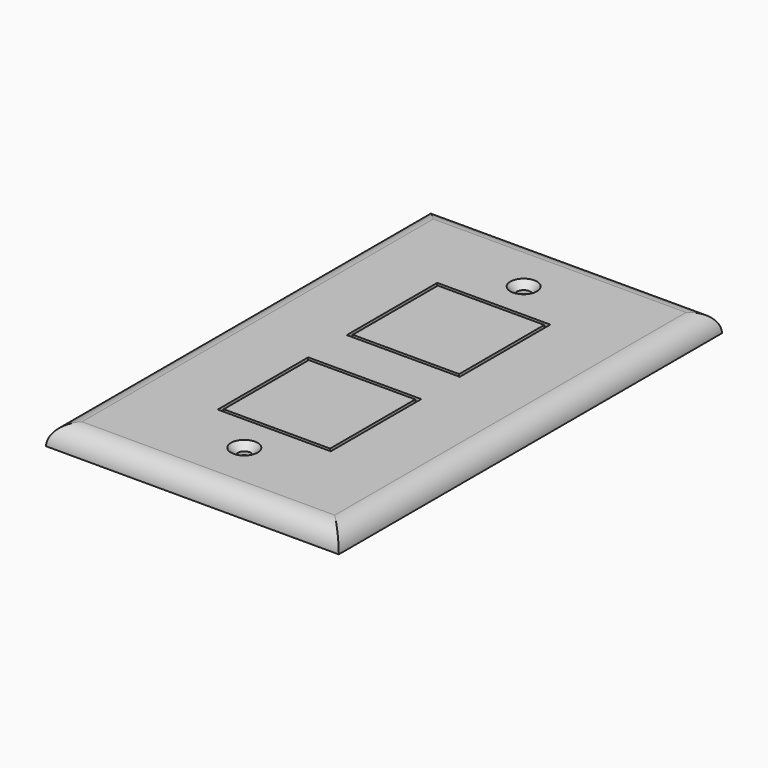
from build123d import *

# Parameters (mm, degrees)
F0_W        = 69.85
F0_H        = 114.3
F0_R        = 1.5875
F1_DEPTH    = 4.7625
F2_R        = 4.76249
F3_SIZE     = 1.5875
F4_W        = 57.15
F4_H        = 101.6
F5_DEPTH    = 2.38125
F6_T1_DEPTH = 101.6
F6_T3_DEPTH = 57.15
F8_DEPTH    = 4.7635
F7_W        = 12.7
F7_H        = 0.79375
F9_DEPTH    = 1.5875
F10_R       = 3.175
F10_R_2     = 1.5875
F11_DEPTH   = 6.35


# Not quite as in the source:
# - a fillet or chamfer that OpenCascade refuses, or shapes differently, is made with other operations: its cross-section is extruded or revolved along the edge and cut away or added
# - a fillet or chamfer is up to 0.001 mm smaller than in the source, because OpenCascade refuses the exact size


with BuildPart() as f1:
    # F0 (on Top) → F1 (new body)
    with BuildSketch(Plane.XY):
        Rectangle(F0_W, F0_H)
        with Locations((0, -41.6687)):
            Circle(F0_R, mode=Mode.SUBTRACT)
        with Locations((0, 41.6687)):
            Circle(F0_R, mode=Mode.SUBTRACT)
    extrude(amount=F1_DEPTH)

    # F2 (radius 4.7625 in the source; OpenCascade refuses exactly that, so slightly less here)
    f2_edges = [f1.edges().sort_by_distance(p)[0] for p in [
        (34.925, 0, 4.7625),
        (0, -57.15, 4.7625),
        (-34.925, 0, 4.7625),
        (0, 57.15, 4.7625),
    ]]
    fillet(f2_edges, radius=F2_R)

    # F3
    f3_edges = [f1.edges().sort_by_distance(p)[0] for p in [
        (-1.5875, 41.6687, 4.7625),
        (-1.5875, -41.6687, 4.7625),
    ]]
    chamfer(f3_edges, length=F3_SIZE)

    # F4 (on face) → F5 (cut)
    with BuildSketch(Plane(origin=(0, 0, 0), x_dir=(1, 0, 0), z_dir=(0, 0, -1))):
        Rectangle(F4_W, F4_H)
    extrude(amount=-F5_DEPTH, mode=Mode.SUBTRACT)

    # F6: fillet of radius 5.08 on 4 edges, made by hand

    # F6_s2 → F6_t1 (join)
    with BuildSketch(Plane.XZ.offset(-50.8)):
        with BuildLine():
            ThreePointArc((24.2711472565, 2.38125), (26.7304916814, 1.74625), (28.575, 0))
            Line((28.575, 0), (28.575, 2.38125))
            Line((28.575, 2.38125), (24.2711472565, 2.38125))
        make_face()
        with BuildLine():
            ThreePointArc((-24.2711472565, 2.38125), (-26.7304916814, 1.74625), (-28.575, 0))
            Line((-28.575, 0), (-28.575, 2.38125))
            Line((-28.575, 2.38125), (-24.2711472565, 2.38125))
        make_face()
    extrude(amount=F6_T1_DEPTH)

    # F6_s4 → F6_t3 (join)
    with BuildSketch(Plane.YZ.offset(-28.575)):
        with BuildLine():
            ThreePointArc((-46.4961472565, 2.38125), (-48.9554916814, 1.74625), (-50.8, 0))
            Line((-50.8, 0), (-50.8, 2.38125))
            Line((-50.8, 2.38125), (-46.4961472565, 2.38125))
        make_face()
        with BuildLine():
            ThreePointArc((46.4961472565, 2.38125), (48.9554916814, 1.74625), (50.8, 0))
            Line((50.8, 0), (50.8, 2.38125))
            Line((50.8, 2.38125), (46.4961472565, 2.38125))
        make_face()
    extrude(amount=F6_T3_DEPTH)

    # F7 (on face) → F8 (cut, through all)
    with BuildSketch(Plane.XY.offset(4.7625)):
        Polygon((-12.7, 31.94685), (12.7, 31.94685), (12.7, 6.54685), (6.35, 6.54685), (6.35, 5.7531), (13.49375, 5.7531), (13.49375, 32.7406), (-13.49375, 32.7406), (-13.49375, 5.7531), (-6.35, 5.7531), (-6.35, 6.54685), (-12.7, 6.54685), align=None)
        Polygon((6.35, -5.7531), (6.35, -6.54685), (12.7, -6.54685), (12.7, -31.94685), (-12.7, -31.94685), (-12.7, -6.54685), (-6.35, -6.54685), (-6.35, -5.7531), (-13.49375, -5.7531), (-13.49375, -32.7406), (13.49375, -32.7406), (13.49375, -5.7531), align=None)
    extrude(amount=-F8_DEPTH, mode=Mode.SUBTRACT)

    # F7 (on face) → F9 (cut)
    with BuildSketch(Plane.XY.offset(4.7625)):
        with Locations((0, 6.149975)):
            Rectangle(F7_W, F7_H)
        with Locations((0, -6.149975)):
            Rectangle(F7_W, F7_H)
    extrude(amount=-F9_DEPTH, mode=Mode.SUBTRACT)

    # F10 (on face) → F11 (join)
    with BuildSketch(Plane(origin=(0, 0, 2.38125), x_dir=(1, 0, 0), z_dir=(0, 0, -1))):
        with Locations((-17.272, 30.6211472565)):
            Circle(F10_R)
        with Locations((-17.272, 30.6211472565)):
            Circle(F10_R_2, mode=Mode.SUBTRACT)
        with Locations((-17.272, -30.5562)):
            Circle(F10_R)
        with Locations((-17.272, -30.6211472565)):
            Circle(F10_R_2, mode=Mode.SUBTRACT)
        with Locations((17.272, 30.6211472565)):
            Circle(F10_R)
        with Locations((17.272, 30.6211472565)):
            Circle(F10_R_2, mode=Mode.SUBTRACT)
        with Locations((17.272, -30.5562)):
            Circle(F10_R)
        with Locations((17.272, -30.6211472565)):
            Circle(F10_R_2, mode=Mode.SUBTRACT)
        Circle(F10_R)
        Circle(F10_R_2, mode=Mode.SUBTRACT)
    extrude(amount=F11_DEPTH)


solid = f1.part
